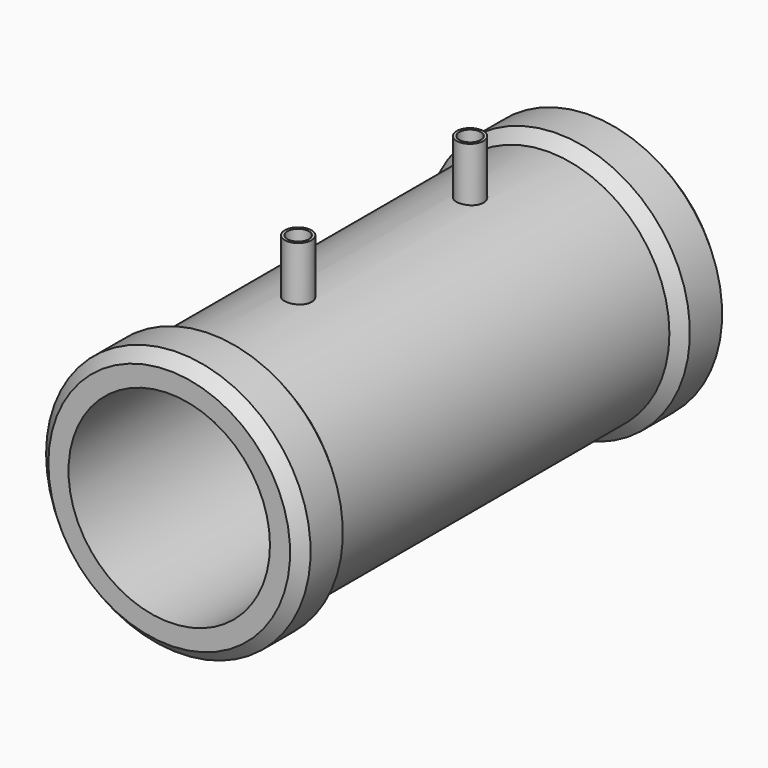
from build123d import *

# Parameters (mm, degrees)
F0_R          = 45
F0_R_2        = 37.5
F1_DEPTH      = 100
F3_R          = 5
F3_R_2        = 4
F4_DEPTH      = 20
F4_DEPTH_BACK = 5


# Not quite as in the source:
# - a pattern or mirror of a feature is missing from the dataset's text; its kind, count and spacing are read off the source's solid


with BuildPart() as f1:
    # F0 (on Front) → F1 (new body, symmetric)
    with BuildSketch(Plane.XZ):
        Circle(F0_R)
        Circle(F0_R_2, mode=Mode.SUBTRACT)
    extrude(amount=F1_DEPTH, both=True)

    # F3 (on offset) → F4 (join, two sides)
    with BuildSketch(Plane.XY.offset(45)) as f4_sk:
        with Locations((0, 40)):
            Circle(F3_R)
        with Locations((0, 40)):
            Circle(F3_R_2, mode=Mode.SUBTRACT)
        with Locations((0, -40)):
            Circle(F3_R)
        with Locations((0, -40)):
            Circle(F3_R_2, mode=Mode.SUBTRACT)
    extrude(amount=F4_DEPTH)
    extrude(f4_sk.sketch, amount=-F4_DEPTH_BACK)

    # F5 (on Top) → F6 (revolve)
    with BuildSketch(Plane.XY):
        Polygon((-49.2426406871, -95.7573593129), (-45, -100), (-45, -76.5147186258), (-49.2426406871, -80.7573593129), align=None)
    f6 = revolve(axis=Axis((0, 11.0722705722, 0), (0, 1, 0)))

    # F6_copies: F6 across plane
    add(f6.mirror(Plane.ZX))


solid = f1.part
